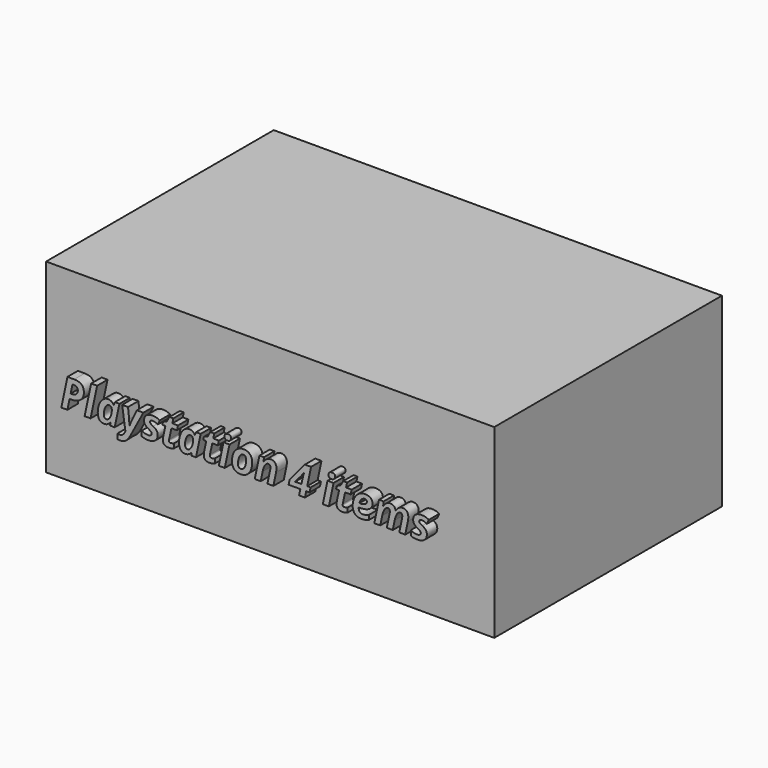
from build123d import *

# Parameters (mm, degrees)
F0_W         = 122.6643398404
F0_H         = 77.8905339539
F1_DEPTH     = 50.8
F2_TEXT_SIZE = 11.1386333659
F3_DEPTH     = 41.91


# Not quite as in the source:
# - Text() gives the source's letters only with a copy of the font that has no kerning and outlines rounded to 1/6400 em; it was checked with that copy


with BuildPart() as f1:
    # F0 (on Top) → F1 (new body)
    with BuildSketch(Plane.XY):
        with Locations((-2.7155689895, 0.5961004645)):
            Rectangle(F0_W, F0_H)
    extrude(amount=F1_DEPTH)

    # F2 (on Front) → F3 (join)
    with BuildSketch(Plane.XZ):
        with Locations((-57.3191848903, 19.3294078712)):
            Text('Playstation 4 items', F2_TEXT_SIZE, font='Open Sans', font_style=FontStyle.BOLDITALIC, text_align=(TextAlign.LEFT, TextAlign.BOTTOM))
    extrude(amount=F3_DEPTH)


solid = f1.part
